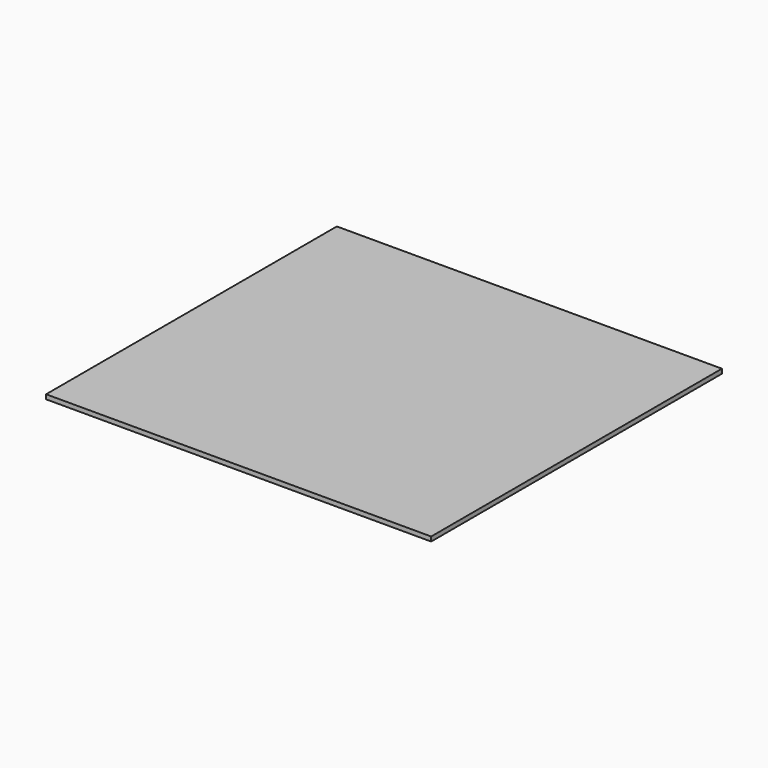
from build123d import *

# Parameters (mm, degrees)
F0_R     = 1.5
F1_DEPTH = 6
F2_R     = 1.5
F3_DEPTH = 5.3
F4_W     = 275.2343043685
F4_H     = 259.7636207938
F4_R     = 1.5
F5_DEPTH = 3.2
F6_DEPTH = 5.3


with BuildPart() as f1:
    # F0 (on Top) → F1 (new body)
    with BuildSketch(Plane.XY):
        Polygon((-118, 140), (-120, 140), (-122, 140), (-125, 137), (-125, 135), (-125, 133), (-105, 113), (-105, 93), (-115, 83), (-115, 45), (-105, 35), (-105, 25), (-115, 15), (-115, -23), (-105, -33), (-105, -53), (-125, -73), (-125, -77), (-122, -80), (-120, -80), (-118, -80), (-93, -55), (63, -55), (88, -80), (90, -80), (92, -80), (95, -77), (95, -73), (75, -53), (55, -33), (55, -13), (75, 7), (85, 17), (85, 43), (75, 53), (55, 73), (55, 93), (95, 133), (95, 136), (95, 137), (92, 140), (88, 140), (65, 117), (63, 115), (-93, 115), align=None)
        with Locations((-119.5, -74.5)):
            Circle(F0_R, mode=Mode.SUBTRACT)
        with Locations((-110, -5)):
            Circle(F0_R, mode=Mode.SUBTRACT)
        with BuildLine():
            ThreePointArc((-101, -20), (-103.8284271247, -18.8284271247), (-105, -16))
            Line((-105, -16), (-105, 7))
            ThreePointArc((-105, 7), (-103.8284271247, 9.8284271247), (-101, 11))
            Line((-101, 11), (-99, 11))
            ThreePointArc((-99, 11), (-96.1715728753, 9.8284271247), (-95, 7))
            Line((-95, 7), (-95, -16))
            ThreePointArc((-95, -16), (-96.1715728753, -18.8284271247), (-99, -20))
            Line((-99, -20), (-101, -20))
        make_face(mode=Mode.SUBTRACT)
        with Locations((-90, -5)):
            Circle(F0_R, mode=Mode.SUBTRACT)
        with Locations((89.5, -74.5)):
            Circle(F0_R, mode=Mode.SUBTRACT)
        Polygon((-43, -5), (13, -5), (53, -45), (-83, -45), align=None, mode=Mode.SUBTRACT)
        with Locations((-15, 9)):
            Circle(F0_R, mode=Mode.SUBTRACT)
        with BuildLine():
            ThreePointArc((75, 17.862876), (73.8284271247, 15.0344488753), (71, 13.862876))
            Line((71, 13.862876), (69, 13.862876))
            ThreePointArc((69, 13.862876), (66.1715728753, 15.0344488753), (65, 17.862876))
            Line((65, 17.862876), (65, 40.862876))
            ThreePointArc((65, 40.862876), (66.1715728753, 43.6913031247), (69, 44.862876))
            Line((69, 44.862876), (71, 44.862876))
            ThreePointArc((71, 44.862876), (73.8284271247, 43.6913031247), (75, 40.862876))
            Line((75, 40.862876), (75, 17.862876))
        make_face(mode=Mode.SUBTRACT)
        with Locations((-110, 65)):
            Circle(F0_R, mode=Mode.SUBTRACT)
        with BuildLine():
            ThreePointArc((-95, 54.007037), (-96.1715728753, 51.1786098753), (-99, 50.007037))
            Line((-99, 50.007037), (-101, 50.007037))
            ThreePointArc((-101, 50.007037), (-103.8284271247, 51.1786098753), (-105, 54.007037))
            Line((-105, 54.007037), (-105, 77.007037))
            ThreePointArc((-105, 77.007037), (-103.8284271247, 79.8354641247), (-101, 81.007037))
            Line((-101, 81.007037), (-99, 81.007037))
            ThreePointArc((-99, 81.007037), (-96.1715728753, 79.8354641247), (-95, 77.007037))
            Line((-95, 77.007037), (-95, 54.007037))
        make_face(mode=Mode.SUBTRACT)
        with Locations((-90, 65)):
            Circle(F0_R, mode=Mode.SUBTRACT)
        Polygon((-95, 25), (-95, 35), (-75, 55), (-55, 55), (-35, 35), (-35, 25), (-55, 5), (-75, 5), align=None, mode=Mode.SUBTRACT)
        with Locations((-119.5, 134.5)):
            Circle(F0_R, mode=Mode.SUBTRACT)
        with Locations((-15, 50)):
            Circle(F0_R, mode=Mode.SUBTRACT)
        Polygon((25, 55), (35, 55), (55, 35), (55, 25), (35, 5), (25, 5), (5, 25), (5, 35), align=None, mode=Mode.SUBTRACT)
        with Locations((60, 30)):
            Circle(F0_R, mode=Mode.SUBTRACT)
        with Locations((80, 30)):
            Circle(F0_R, mode=Mode.SUBTRACT)
        Polygon((53, 105), (25, 77), (23, 75), (13, 65), (-43, 65), (-83, 105), align=None, mode=Mode.SUBTRACT)
        with Locations((89.5, 134.5)):
            Circle(F0_R, mode=Mode.SUBTRACT)
    extrude(amount=F1_DEPTH)


with BuildPart() as f3:
    # F2 (on face) → F3 (new body)
    with BuildSketch(Plane.XY.offset(6)):
        Polygon((-118, 131.9019237886), (-116.5, 134.5), (-118, 137.0980762114), (-121, 137.0980762114), (-122.5, 134.5), (-121, 131.9019237886), align=None)
        with Locations((-119.5, 134.5)):
            Circle(F2_R, mode=Mode.SUBTRACT)
    extrude(amount=F3_DEPTH)

    # F4 (on face) → F5 (join)
    with BuildSketch(Plane.XY.offset(11.3)):
        with Locations((-14.0173770487, 28.0120261014)):
            Rectangle(F4_W, F4_H)
        Polygon((-116.5, 134.5), (-118, 131.9019237886), (-121, 131.9019237886), (-122.5, 134.5), (-121, 137.0980762114), (-118, 137.0980762114), align=None, mode=Mode.SUBTRACT)
        Polygon((-121, 131.9019237886), (-118, 131.9019237886), (-116.5, 134.5), (-118, 137.0980762114), (-121, 137.0980762114), (-122.5, 134.5), align=None)
        with Locations((-119.5, 134.5)):
            Circle(F4_R, mode=Mode.SUBTRACT)
        with Locations((-119.5, 134.5)):
            Circle(F4_R)
    extrude(amount=F5_DEPTH)

    # F2 (on face) → F6 (join, through all)
    with BuildSketch(Plane.XY.offset(6)):
        Polygon((-118, -77.0980762114), (-116.5, -74.5), (-118, -71.9019237886), (-121, -71.9019237886), (-122.5, -74.5), (-121, -77.0980762114), align=None)
        with Locations((-119.5, -74.5)):
            Circle(F2_R, mode=Mode.SUBTRACT)
        Polygon((-13.5, 6.4019237886), (-12, 9), (-13.5, 11.5980762114), (-16.5, 11.5980762114), (-18, 9), (-16.5, 6.4019237886), align=None)
        with Locations((-15, 9)):
            Circle(F2_R, mode=Mode.SUBTRACT)
        Polygon((-13.5, 47.4019237886), (-12, 50), (-13.5, 52.5980762114), (-16.5, 52.5980762114), (-18, 50), (-16.5, 47.4019237886), align=None)
        with Locations((-15, 50)):
            Circle(F2_R, mode=Mode.SUBTRACT)
        Polygon((88, 137.0980762114), (86.5, 134.5), (88, 131.9019237886), (91, 131.9019237886), (92.5, 134.5), (91, 137.0980762114), align=None)
        with Locations((89.5, 134.5)):
            Circle(F2_R, mode=Mode.SUBTRACT)
        Polygon((91, -77.0980762114), (92.5, -74.5), (91, -71.9019237886), (88, -71.9019237886), (86.5, -74.5), (88, -77.0980762114), align=None)
        with Locations((89.5, -74.5)):
            Circle(F2_R, mode=Mode.SUBTRACT)
    extrude(amount=F6_DEPTH)


solid = Compound([f1.part, f3.part])
